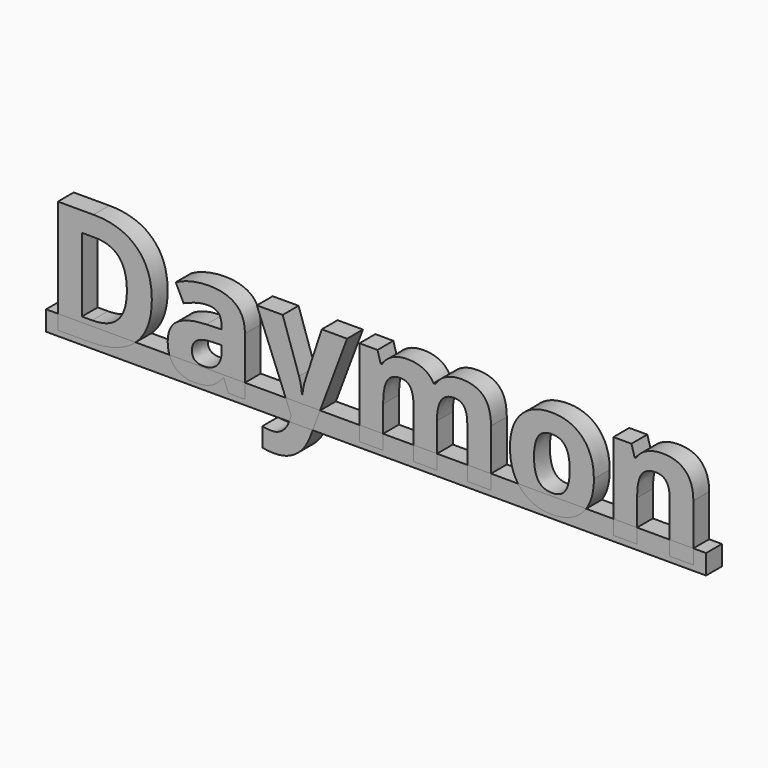
from build123d import *

# Parameters (mm, degrees)
F0_TEXT_SIZE = 24.0312406128
F1_DEPTH     = 3
F2_W         = 100
F2_H         = 3
F3_DEPTH     = 3
F4_DEPTH     = 3


# Not quite as in the source:
# - Text() gives the source's letters only with a copy of the font that has no kerning and outlines rounded to 1/6400 em; it was checked with that copy


with BuildPart() as f1:
    # F0 (on Front) → F1 (new body)
    with BuildSketch(Plane.XZ):
        with Locations((-50, 0)):
            Text('Daymon', F0_TEXT_SIZE, font='Open Sans', font_style=FontStyle.BOLD, text_align=(TextAlign.LEFT, TextAlign.BOTTOM))
    extrude(amount=F1_DEPTH)

    # F2 (on Front) → F3 (join)
    with BuildSketch(Plane.XZ):
        with Locations((0.3723084927, 0.7102387156)):
            Rectangle(F2_W, F2_H)
    extrude(amount=F3_DEPTH)

    # F2 (on Front) → F4 (join)
    with BuildSketch(Plane.XZ):
        with Locations((0.3723084927, 0.7102387156)):
            Rectangle(F2_W, F2_H)
    extrude(amount=F4_DEPTH)


solid = f1.part
